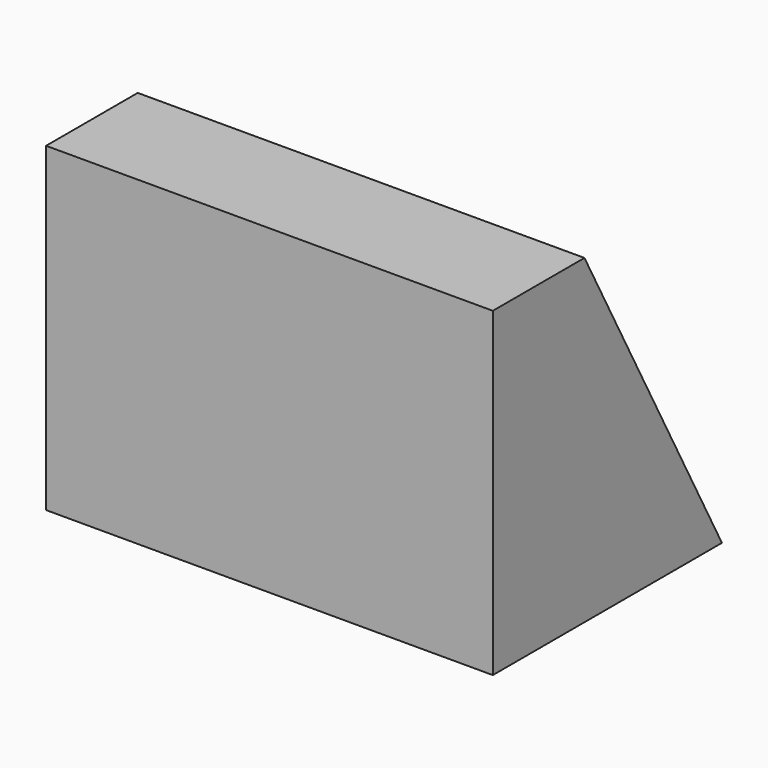
from build123d import *

# Parameters (mm, degrees)
F4_W     = 390
F4_H     = 250
F5_DEPTH = 280
F6_SIZE2 = 149.99999
F6_SIZE  = 279.99999
F7_T     = 8


# Not quite as in the source:
# - a fillet or chamfer is up to 0.001 mm smaller than in the source, because OpenCascade refuses the exact size
# - a shell that OpenCascade refuses in one call is made with other operations: the cavity is built on its own and cut out


with BuildPart() as f5:
    # F4 (on Top) → F5 (new body)
    with BuildSketch(Plane.XY):
        with Locations((9.861856699, -53.0331014672)):
            Rectangle(F4_W, F4_H)
    extrude(amount=F5_DEPTH)

    # F6 (size 280 and 150 in the source; OpenCascade refuses exactly that, so slightly less here)
    f6_edges = [f5.edges().sort_by_distance(p)[0] for p in [
        (9.861857, 71.966899, 280),
    ]]
    f6_side = f5.faces().sort_by_distance((9.861857, 71.966899, 140))[0]
    chamfer(f6_edges, length=F6_SIZE, length2=F6_SIZE2, reference=f6_side)

    # F7: shell of thickness 8, made by hand


with BuildPart() as f7_core1:
    # F7_t2: copy of F5
    add(f5.part)

    # the walls: a layer under each face that stays
    f7_faces = [f7_core1.faces().sort_by_distance(p)[0] for p in [
        (-185.138143301, -53.0331014672, 140),
        (9.861856699, 71.9668985328, 5e-06),
        (9.861856699, -3.0330964672, 140.000005),
        (9.861856699, -128.0330964672, 280),
        (9.861856699, -178.0331014672, 140),
        (204.861856699, -53.0331014672, 140),
    ]]
    thicken(f7_faces, amount=-F7_T, mode=Mode.SUBTRACT)


with BuildPart() as f5_1:
    add(f5.part)

    # what is left inside the walls is the cavity
    f7_cavity = [f7_core1.part.solids().sort_by_distance(p)[0] for p in [
        (9.861857, 14.249313, 90.628889),
    ]]
    add(f7_cavity, mode=Mode.SUBTRACT)


solid = f5_1.part
